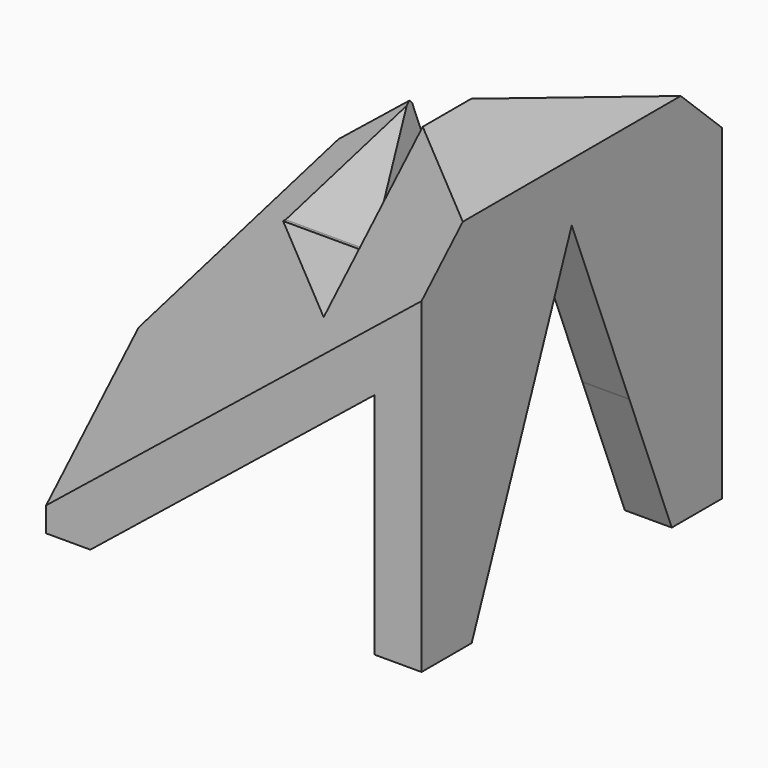
from build123d import *

# Parameters (mm, degrees)
F0_W           = 80
F0_H           = 80
F1_DEPTH       = 80
F3_DEPTH       = 86.9
F4_W           = 8
F4_H           = 80
F5_DEPTH       = 25
F6_W           = 30
F6_H           = 25
F7_DEPTH       = 25
F9_DEPTH       = 50.3
F11_W          = 223.7579002976
F11_H          = 231.868326664
F12_DEPTH      = 25
F13_W          = 207.2095647454
F13_H          = 262.1310725808
F14_DEPTH      = 25
F16_DEPTH      = 127.5
F18_DEPTH      = 40.001
F18_DEPTH_BACK = 40.001


# Not quite as in the source:
# - a feature of the source that left no trace in its solid (it failed there, or was rolled back) is left out


with BuildPart() as f1:
    # F0 (on Top) → F1 (new body)
    with BuildSketch(Plane.XY):
        Rectangle(F0_W, F0_H)
    extrude(amount=F1_DEPTH)

    # F2 (on face) → F3 (cut)
    with BuildSketch(Plane.XZ.offset(40)):
        Polygon((-40, 28.6014117301), (0, 80), (-40, 80), align=None)
    extrude(amount=-F3_DEPTH, mode=Mode.SUBTRACT)

    # F4 (on face) → F5 (cut)
    with BuildSketch(Plane.XY.offset(80)):
        with Locations((9.4103766605, 0)):
            Rectangle(F4_W, F4_H)
    extrude(amount=-F5_DEPTH, mode=Mode.SUBTRACT)

    # F6 (on face) → F7 (cut)
    with BuildSketch(Plane.YZ.offset(5.4103766605)):
        with Locations((-25, 67.5)):
            Rectangle(F6_W, F6_H)
        with Locations((25, 67.5)):
            Rectangle(F6_W, F6_H)
    extrude(amount=-F7_DEPTH, mode=Mode.SUBTRACT)

    # F8 (on face) → F9 (cut)
    with BuildSketch(Plane(origin=(-40, 0, 0), x_dir=(0, -1, 0), z_dir=(-1, 0, 0))):
        Polygon((-10.1708276197, 55.0271123648), (0, 80.8042436838), (10.1708276197, 55.0271123648), (61.0520653427, 55.0271123648), (61.0520653427, 88.9606252313), (0, 88.9606252313), (-61.0520653427, 88.9606252313), (-61.0520653427, 55.0271123648), align=None)
    extrude(amount=-F9_DEPTH, mode=Mode.SUBTRACT)

    # F11 (on face) → F12 (cut)
    with BuildSketch(Plane(origin=(-23.8023577799, -28.0559598365, 29.5937245096), x_dir=(0.8636441264, -0.3468224195, 0.3658319728), z_dir=(-0.5041019966, -0.5941875801, 0.6267553723))):
        with Locations((27.8940685093, 6.7206919193)):
            Rectangle(F11_W, F11_H)
    extrude(amount=F12_DEPTH, mode=Mode.SUBTRACT)

    # F13 (on face) → F14 (cut)
    with BuildSketch(Plane(origin=(-23.8023577799, 28.0559598365, 29.5937245096), x_dir=(0.8636441264, 0.3468224195, 0.3658319728), z_dir=(-0.5041019966, 0.5941875801, 0.6267553723))):
        with Locations((8.8918171823, -6.4797215164)):
            Rectangle(F13_W, F13_H)
    extrude(amount=F14_DEPTH, mode=Mode.SUBTRACT)

    # F15 (on face) → F16 (cut)
    with BuildSketch(Plane.XZ.offset(40)):
        Polygon((30, 0), (30, 48.7106099482), (-30.5624192708, 0), align=None)
    extrude(amount=-F16_DEPTH, mode=Mode.SUBTRACT)

    # F17 (on Right) → F18 (cut, two sides)
    with BuildSketch(Plane.YZ) as f18_sk:
        Polygon((15.2906342708, 28.7791552365), (0, 67.5320180601), (-15.3222406511, 28.6990514489), (-15.3607661463, 28.6014117301), (15.3607661463, 28.6014117301), align=None)
        Polygon((26.6459640524, 0), (15.3607661463, 28.6014117301), (-15.3607661463, 28.6014117301), (-26.6459640524, 0), align=None)
    extrude(amount=-F18_DEPTH, mode=Mode.SUBTRACT)
    extrude(f18_sk.sketch, amount=F18_DEPTH_BACK, mode=Mode.SUBTRACT)


solid = f1.part
